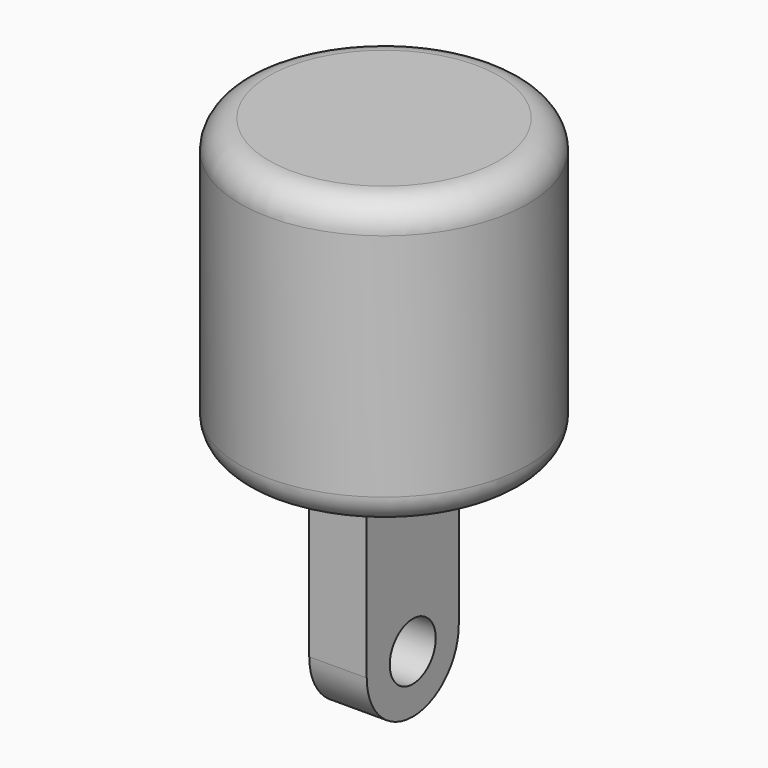
from build123d import *

# Parameters (mm, degrees)
F0_R     = 25
F1_DEPTH = 50
F2_W     = 10
F2_H     = 20
F3_DEPTH = 40
F6_R     = 9.99999
F7_R     = 5
F5_D     = 10


# Not quite as in the source:
# - a fillet or chamfer is up to 0.001 mm smaller than in the source, because OpenCascade refuses the exact size


with BuildPart() as f1:
    # F0 (on Top) → F1 (new body)
    with BuildSketch(Plane.XY):
        Circle(F0_R)
    extrude(amount=F1_DEPTH)

    # F2 (on face) → F3 (join)
    with BuildSketch(Plane(origin=(0, 0, 0), x_dir=(1, 0, 0), z_dir=(0, 0, -1))):
        Rectangle(F2_W, F2_H)
    extrude(amount=F3_DEPTH)

    # F6 (radius 10 in the source; OpenCascade refuses exactly that, so slightly less here)
    f6_edges = [f1.edges().sort_by_distance(p)[0] for p in [
        (0, 10, -40),
        (0, -10, -40),
    ]]
    fillet(f6_edges, radius=F6_R)

    # F7
    f7_edges = [f1.edges().sort_by_distance(p)[0] for p in [
        (-25, 0, 50),
        (-25, 0, 0),
        (-5, 0, 0),
        (0, -10, 0),
        (5, 0, 0),
        (0, 10, 0),
    ]]
    fillet(f7_edges, radius=F7_R)

    # F5 (through all)
    with Locations(Plane(origin=(-5, 0, 0), x_dir=(0, -1, 0), z_dir=(-1, 0, 0))):
        with Locations((0, -30)):
            Hole(F5_D / 2)


solid = f1.part
